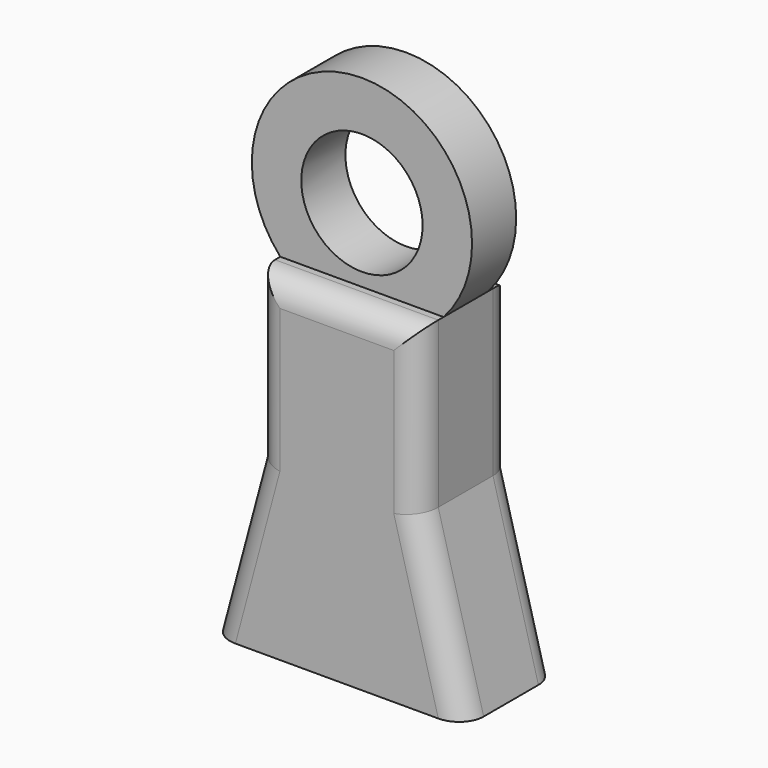
from build123d import *

# Parameters (mm, degrees)
F0_R     = 8.485
F0_R_2   = 4.675
F1_DEPTH = 2.125
F2_W     = 12.5812107759
F2_H     = 12.7
F3_DEPTH = 4.539996
F5_DEPTH = 2.0625
F6_R     = 2.06249
F7_R     = 1.905


# Not quite as in the source:
# - a fillet or chamfer is up to 0.001 mm smaller than in the source, because OpenCascade refuses the exact size


with BuildPart() as f1:
    # F0 (on Front) → F1 (new body, symmetric)
    with BuildSketch(Plane.XZ):
        Circle(F0_R)
        Circle(F0_R_2, mode=Mode.SUBTRACT)
    extrude(amount=F1_DEPTH, both=True)

    # F2 (on Front) → F3 (join, symmetric)
    with BuildSketch(Plane.XZ):
        Polygon((-6.2906053879, -18.3941644561), (-9.7885362858, -31.4486202883), (9.7885362858, -31.4486202883), (6.2906053879, -18.3941644561), align=None)
        with Locations((0, -12.0441644561)):
            Rectangle(F2_W, F2_H)
    extrude(amount=F3_DEPTH, both=True)

    # F4 (on Front) → F5 (cut, symmetric)
    with BuildSketch(Plane.XZ):
        Polygon((4.22592549, -20.5024805709), (0.2414814566, -21.5701091319), (2.8884205433, -31.4486202883), (7.1589347875, -31.4486202883), align=None)
        Polygon((-0.2414814566, -21.5701091319), (-4.22592549, -20.5024805709), (-6.8555269883, -30.3162869659), (-7.1589347875, -31.4486202883), (-2.8884205433, -31.4486202883), align=None)
    extrude(amount=F5_DEPTH, both=True, mode=Mode.SUBTRACT)

    # F6 (radius 2.0625 in the source; OpenCascade refuses exactly that, so slightly less here)
    f6_edges = [f1.edges().sort_by_distance(p)[0] for p in [
        (-5.69243, -2.0625, -25.97555),
        (1.564951, -2.0625, -26.509365),
        (5.69243, -2.0625, -25.97555),
        (-1.564951, -2.0625, -26.509365),
        (5.69243, 2.0625, -25.97555),
        (-1.564951, 2.0625, -26.509365),
        (-5.69243, 2.0625, -25.97555),
        (1.564951, 2.0625, -26.509365),
    ]]
    fillet(f6_edges, radius=F6_R)

    # F7
    f7_edges = [f1.edges().sort_by_distance(p)[0] for p in [
        (-8.039571, -4.539996, -24.921392),
        (-6.290605, -4.539996, -12.044164),
        (-6.290605, 4.539996, -12.044164),
        (-8.039571, 4.539996, -24.921392),
        (8.039571, -4.539996, -24.921392),
        (6.290605, -4.539996, -12.044164),
        (8.039571, 4.539996, -24.921392),
        (6.290605, 4.539996, -12.044164),
        (0, 4.539996, -5.694164),
        (0, -4.539996, -5.694164),
    ]]
    fillet(f7_edges, radius=F7_R)


solid = f1.part
